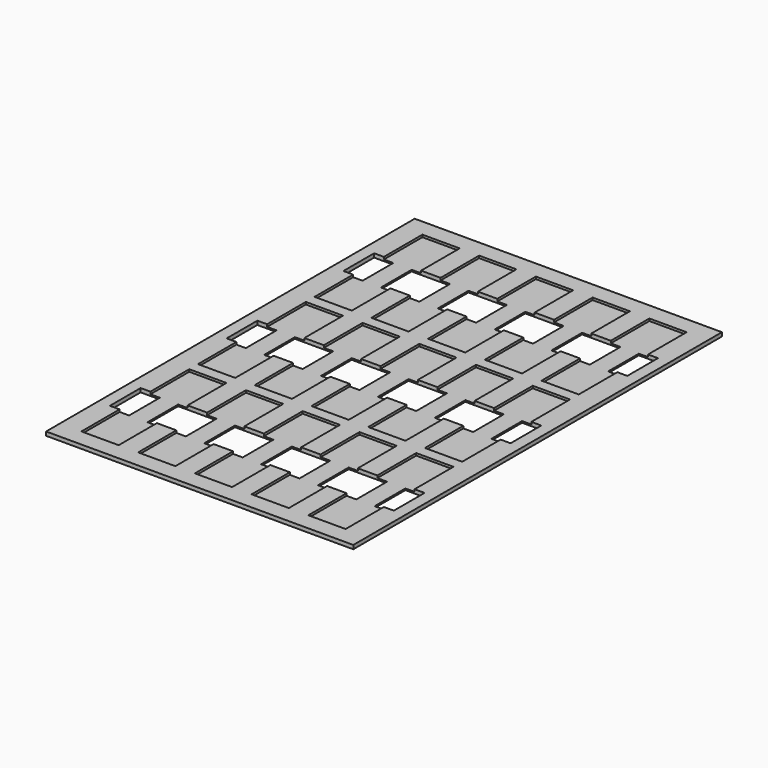
from build123d import *

# Parameters (mm, degrees)
F0_W         = 400
F0_H         = 600
F1_DEPTH     = 2
F2_W         = 400
F2_H         = 600
F2_W_2       = 48.5
F2_H_2       = 175.5
F3_DEPTH     = 3
F4_W         = 50
F4_H         = 50
F4_W_2       = 25
F5_DEPTH     = 25
F6_T         = 2
F6_T3_DEPTH  = 7
F6_T5_DEPTH  = 52.5
F6_T7_DEPTH  = 66.25
F6_T9_DEPTH  = 6
F6_T11_DEPTH = 52.5
F6_T13_DEPTH = 52.5
F6_T15_DEPTH = 52.5
F6_T17_DEPTH = 52.5
F6_T19_DEPTH = 9
F6_T21_DEPTH = 67.25
F6_T23_DEPTH = 66.5
F6_T25_DEPTH = 67
F6_T27_DEPTH = 66.75
F6_T29_DEPTH = 66.75


# Not quite as in the source:
# - a shell that OpenCascade refuses in one call is made with other operations: the cavity is built on its own and cut out


with BuildPart() as f1:
    # F0 (on Top) → F1 (new body)
    with BuildSketch(Plane.XY):
        Rectangle(F0_W, F0_H)
    extrude(amount=F1_DEPTH)

    # F2 (on face) → F3 (join)
    with BuildSketch(Plane.XY.offset(2)):
        Rectangle(F2_W, F2_H)
        with Locations((-147.75, -189.75)):
            Rectangle(F2_W_2, F2_H_2, mode=Mode.SUBTRACT)
        with Locations((-73.875, -189.75)):
            Rectangle(F2_W_2, F2_H_2, mode=Mode.SUBTRACT)
        with Locations((0, -189.75)):
            Rectangle(F2_W_2, F2_H_2, mode=Mode.SUBTRACT)
        with Locations((73.875, -189.75)):
            Rectangle(F2_W_2, F2_H_2, mode=Mode.SUBTRACT)
        with Locations((147.75, -189.75)):
            Rectangle(F2_W_2, F2_H_2, mode=Mode.SUBTRACT)
        with Locations((-147.75, 0)):
            Rectangle(F2_W_2, F2_H_2, mode=Mode.SUBTRACT)
        with Locations((-73.875, 0)):
            Rectangle(F2_W_2, F2_H_2, mode=Mode.SUBTRACT)
        with Locations((-147.75, 189.75)):
            Rectangle(F2_W_2, F2_H_2, mode=Mode.SUBTRACT)
        with Locations((-73.875, 189.75)):
            Rectangle(F2_W_2, F2_H_2, mode=Mode.SUBTRACT)
        Rectangle(F2_W_2, F2_H_2, mode=Mode.SUBTRACT)
        with Locations((73.875, 0)):
            Rectangle(F2_W_2, F2_H_2, mode=Mode.SUBTRACT)
        with Locations((147.75, 0)):
            Rectangle(F2_W_2, F2_H_2, mode=Mode.SUBTRACT)
        with Locations((0, 189.75)):
            Rectangle(F2_W_2, F2_H_2, mode=Mode.SUBTRACT)
        with Locations((73.875, 189.75)):
            Rectangle(F2_W_2, F2_H_2, mode=Mode.SUBTRACT)
        with Locations((147.75, 189.75)):
            Rectangle(F2_W_2, F2_H_2, mode=Mode.SUBTRACT)
    extrude(amount=F3_DEPTH)

    # F4 (on face) → F5 (cut)
    with BuildSketch(Plane.XY.offset(5)):
        with Locations((-110.8125, 189.75)):
            Rectangle(F4_W, F4_H)
        with Locations((-110.8125, -0.25)):
            Rectangle(F4_W, F4_H)
        with Locations((-110.8125, -190.25)):
            Rectangle(F4_W, F4_H)
        with Locations((-36.8125, 189.75)):
            Rectangle(F4_W, F4_H)
        with Locations((-36.8125, -0.25)):
            Rectangle(F4_W, F4_H)
        with Locations((-36.8125, -190.25)):
            Rectangle(F4_W, F4_H)
        with Locations((37.1875, 189.75)):
            Rectangle(F4_W, F4_H)
        with Locations((37.1875, -0.25)):
            Rectangle(F4_W, F4_H)
        with Locations((37.1875, -190.25)):
            Rectangle(F4_W, F4_H)
        with Locations((111.1875, 189.75)):
            Rectangle(F4_W, F4_H)
        with Locations((111.1875, -0.25)):
            Rectangle(F4_W, F4_H)
        with Locations((111.1875, -190.25)):
            Rectangle(F4_W, F4_H)
        with Locations((-172.1875, 189.75)):
            Rectangle(F4_W_2, F4_H)
        with Locations((-172.1875, -0.25)):
            Rectangle(F4_W_2, F4_H)
        with Locations((172.5, 189.75)):
            Rectangle(F4_W_2, F4_H)
        with Locations((172.5, -0.25)):
            Rectangle(F4_W_2, F4_H)
        with Locations((-172.1875, -190.25)):
            Rectangle(F4_W_2, F4_H)
        with Locations((172.5, -190.25)):
            Rectangle(F4_W_2, F4_H)
    extrude(amount=-F5_DEPTH, mode=Mode.SUBTRACT)

    # F6: shell of thickness 2, made by hand


with BuildPart() as f6_core1:
    # F6_t2: copy of F1
    add(f1.part)

    # the walls: a layer under each face that stays
    f6_faces = [f6_core1.faces().sort_by_distance(p)[0] for p in [
        (0, -300, 2.5),
        (-200, 0, 2.5),
        (-114.2857142857, -257.1428571429, 5),
        (200, 0, 2.5),
        (0, 300, 2.5),
        (-147.75, -277.5, 3.5),
        (-123.5, -246.375, 3.5),
        (-110.8125, -215.25, 2.5),
        (-98.125, -246.375, 3.5),
        (-73.875, -277.5, 3.5),
        (-49.625, -246.375, 3.5),
        (-36.8125, -215.25, 2.5),
        (-24.25, -246.375, 3.5),
        (0, -277.5, 3.5),
        (24.25, -246.375, 3.5),
        (37.1875, -215.25, 2.5),
        (49.625, -246.375, 3.5),
        (73.875, -277.5, 3.5),
        (98.125, -246.375, 3.5),
        (111.1875, -215.25, 2.5),
        (123.5, -246.375, 3.5),
        (147.75, -277.5, 3.5),
        (172, -246.375, 3.5),
        (172.5, -215.25, 2.5),
        (185, -190.25, 2.5),
        (172.5, -165.25, 2.5),
        (172, -133.625, 3.5),
        (147.75, -102, 3.5),
        (123.5, -133.625, 3.5),
        (111.1875, -165.25, 2.5),
        (98.125, -133.625, 3.5),
        (73.875, -102, 3.5),
        (49.625, -133.625, 3.5),
        (37.1875, -165.25, 2.5),
        (24.25, -133.625, 3.5),
        (0, -102, 3.5),
        (-24.25, -133.625, 3.5),
        (-36.8125, -165.25, 2.5),
        (-49.625, -133.625, 3.5),
        (-73.875, -102, 3.5),
        (-98.125, -133.625, 3.5),
        (-110.8125, -165.25, 2.5),
        (-123.5, -133.625, 3.5),
        (-147.75, -102, 3.5),
        (-172, -133.625, 3.5),
        (-172.1875, -165.25, 2.5),
        (-184.6875, -190.25, 2.5),
        (-172.1875, -215.25, 2.5),
        (-172, -246.375, 3.5),
        (-147.75, -87.75, 3.5),
        (-123.5, -56.5, 3.5),
        (-110.8125, -25.25, 2.5),
        (-98.125, -56.5, 3.5),
        (-73.875, -87.75, 3.5),
        (-49.625, -56.5, 3.5),
        (-36.8125, -25.25, 2.5),
        (-24.25, -56.5, 3.5),
        (0, -87.75, 3.5),
        (24.25, -56.5, 3.5),
        (37.1875, -25.25, 2.5),
        (49.625, -56.5, 3.5),
        (73.875, -87.75, 3.5),
        (98.125, -56.5, 3.5),
        (111.1875, -25.25, 2.5),
        (123.5, -56.5, 3.5),
        (147.75, -87.75, 3.5),
        (172, -56.5, 3.5),
        (172.5, -25.25, 2.5),
        (185, -0.25, 2.5),
        (172.5, 24.75, 2.5),
        (172, 56.25, 3.5),
        (147.75, 87.75, 3.5),
        (123.5, 56.25, 3.5),
        (111.1875, 24.75, 2.5),
        (98.125, 56.25, 3.5),
        (73.875, 87.75, 3.5),
        (49.625, 56.25, 3.5),
        (37.1875, 24.75, 2.5),
        (24.25, 56.25, 3.5),
        (0, 87.75, 3.5),
        (-24.25, 56.25, 3.5),
        (-36.8125, 24.75, 2.5),
        (-49.625, 56.25, 3.5),
        (-73.875, 87.75, 3.5),
        (-98.125, 56.25, 3.5),
        (-110.8125, 24.75, 2.5),
        (-123.5, 56.25, 3.5),
        (-147.75, 87.75, 3.5),
        (-172, 56.25, 3.5),
        (-172.1875, 24.75, 2.5),
        (-184.6875, -0.25, 2.5),
        (-172.1875, -25.25, 2.5),
        (-172, -56.5, 3.5),
        (-147.75, 102, 3.5),
        (-123.5, 133.375, 3.5),
        (-110.8125, 164.75, 2.5),
        (-98.125, 133.375, 3.5),
        (-73.875, 102, 3.5),
        (-49.625, 133.375, 3.5),
        (-36.8125, 164.75, 2.5),
        (-24.25, 133.375, 3.5),
        (0, 102, 3.5),
        (24.25, 133.375, 3.5),
        (37.1875, 164.75, 2.5),
        (49.625, 133.375, 3.5),
        (73.875, 102, 3.5),
        (98.125, 133.375, 3.5),
        (111.1875, 164.75, 2.5),
        (123.5, 133.375, 3.5),
        (147.75, 102, 3.5),
        (172, 133.375, 3.5),
        (172.5, 164.75, 2.5),
        (185, 189.75, 2.5),
        (172.5, 214.75, 2.5),
        (172, 246.125, 3.5),
        (147.75, 277.5, 3.5),
        (123.5, 246.125, 3.5),
        (111.1875, 214.75, 2.5),
        (98.125, 246.125, 3.5),
        (73.875, 277.5, 3.5),
        (49.625, 246.125, 3.5),
        (37.1875, 214.75, 2.5),
        (24.25, 246.125, 3.5),
        (0, 277.5, 3.5),
        (-24.25, 246.125, 3.5),
        (-36.8125, 214.75, 2.5),
        (-49.625, 246.125, 3.5),
        (-73.875, 277.5, 3.5),
        (-98.125, 246.125, 3.5),
        (-110.8125, 214.75, 2.5),
        (-123.5, 246.125, 3.5),
        (-147.75, 277.5, 3.5),
        (-172, 246.125, 3.5),
        (-172.1875, 214.75, 2.5),
        (-184.6875, 189.75, 2.5),
        (-172.1875, 164.75, 2.5),
        (-172, 133.375, 3.5),
        (-159.6875, -190.25, 1),
        (-85.8125, -190.25, 1),
        (-135.8125, -190.25, 1),
        (-11.8125, -190.25, 1),
        (-61.8125, -190.25, 1),
        (62.1875, -190.25, 1),
        (12.1875, -190.25, 1),
        (136.1875, -190.25, 1),
        (86.1875, -190.25, 1),
        (160, -190.25, 1),
        (-159.6875, -0.25, 1),
        (-85.8125, -0.25, 1),
        (-135.8125, -0.25, 1),
        (-11.8125, -0.25, 1),
        (-61.8125, -0.25, 1),
        (-159.6875, 189.75, 1),
        (-135.8125, 189.75, 1),
        (-85.8125, 189.75, 1),
        (-11.8125, 189.75, 1),
        (-61.8125, 189.75, 1),
        (62.1875, -0.25, 1),
        (12.1875, -0.25, 1),
        (136.1875, -0.25, 1),
        (86.1875, -0.25, 1),
        (160, -0.25, 1),
        (62.1875, 189.75, 1),
        (12.1875, 189.75, 1),
        (136.1875, 189.75, 1),
        (86.1875, 189.75, 1),
        (160, 189.75, 1),
        (-147.75, -189.75, 2),
        (-73.875, -189.75, 2),
        (0, -189.75, 2),
        (73.875, -189.75, 2),
        (147.75, -189.75, 2),
        (-147.75, 0, 2),
        (-73.875, 0, 2),
        (0, 0, 2),
        (73.875, 0, 2),
        (147.75, 0, 2),
        (-147.75, 189.75, 2),
        (-73.875, 189.75, 2),
        (0, 189.75, 2),
        (73.875, 189.75, 2),
        (147.75, 189.75, 2),
    ]]
    thicken(f6_faces, amount=-F6_T, mode=Mode.SUBTRACT)

    # F6_s4 → F6_t3 (cut)
    with BuildSketch(Plane.XY):
        Polygon((-123.52, -277.48), (-123.5, -279.5), (-121.5, -279.5), (-121.5, -277.5), align=None)
        Polygon((-171.98, -277.48), (-172, -279.5), (-174, -279.5), (-174, -277.5), align=None)
        Polygon((-98.105, -277.48), (-100.125, -277.5), (-100.125, -279.5), (-98.125, -279.5), align=None)
        Polygon((-49.645, -277.48), (-49.625, -279.5), (-47.625, -279.5), (-47.625, -277.5), align=None)
        Polygon((-24.23, -277.48), (-26.25, -277.5), (-26.25, -279.5), (-24.25, -279.5), align=None)
        Polygon((24.23, -277.48), (24.25, -279.5), (26.25, -279.5), (26.25, -277.5), align=None)
        Polygon((49.645, -277.48), (47.625, -277.5), (47.625, -279.5), (49.625, -279.5), align=None)
        Polygon((98.105, -277.48), (98.125, -279.5), (100.125, -279.5), (100.125, -277.5), align=None)
        Polygon((123.52, -277.48), (121.5, -277.5), (121.5, -279.5), (123.5, -279.5), align=None)
        Polygon((171.98, -277.48), (172, -279.5), (174, -279.5), (174, -277.5), align=None)
        Polygon((171.98, -102.02), (174, -102), (174, -100), (172, -100), align=None)
        Polygon((123.52, -102.02), (123.5, -100), (121.5, -100), (121.5, -102), align=None)
        Polygon((98.105, -102.02), (100.125, -102), (100.125, -100), (98.125, -100), align=None)
        Polygon((49.645, -102.02), (49.625, -100), (47.625, -100), (47.625, -102), align=None)
        Polygon((24.23, -102.02), (26.25, -102), (26.25, -100), (24.25, -100), align=None)
        Polygon((-24.23, -102.02), (-24.25, -100), (-26.25, -100), (-26.25, -102), align=None)
        Polygon((-49.645, -102.02), (-47.625, -102), (-47.625, -100), (-49.625, -100), align=None)
        Polygon((-98.105, -102.02), (-98.125, -100), (-100.125, -100), (-100.125, -102), align=None)
        Polygon((-123.52, -102.02), (-121.5, -102), (-121.5, -100), (-123.5, -100), align=None)
        Polygon((-171.98, -102.02), (-172, -100), (-174, -100), (-174, -102), align=None)
        Polygon((-123.52, -87.73), (-123.5, -89.75), (-121.5, -89.75), (-121.5, -87.75), align=None)
        Polygon((-171.98, -87.73), (-172, -89.75), (-174, -89.75), (-174, -87.75), align=None)
        Polygon((-98.105, -87.73), (-100.125, -87.75), (-100.125, -89.75), (-98.125, -89.75), align=None)
        Polygon((-49.645, -87.73), (-49.625, -89.75), (-47.625, -89.75), (-47.625, -87.75), align=None)
        Polygon((-24.23, -87.73), (-26.25, -87.75), (-26.25, -89.75), (-24.25, -89.75), align=None)
        Polygon((24.23, -87.73), (24.25, -89.75), (26.25, -89.75), (26.25, -87.75), align=None)
        Polygon((49.645, -87.73), (47.625, -87.75), (47.625, -89.75), (49.625, -89.75), align=None)
        Polygon((98.105, -87.73), (98.125, -89.75), (100.125, -89.75), (100.125, -87.75), align=None)
        Polygon((123.52, -87.73), (121.5, -87.75), (121.5, -89.75), (123.5, -89.75), align=None)
        Polygon((171.98, -87.73), (172, -89.75), (174, -89.75), (174, -87.75), align=None)
        Polygon((171.98, 87.73), (174, 87.75), (174, 89.75), (172, 89.75), align=None)
        Polygon((123.52, 87.73), (123.5, 89.75), (121.5, 89.75), (121.5, 87.75), align=None)
        Polygon((98.105, 87.73), (100.125, 87.75), (100.125, 89.75), (98.125, 89.75), align=None)
        Polygon((49.645, 87.73), (49.625, 89.75), (47.625, 89.75), (47.625, 87.75), align=None)
        Polygon((24.23, 87.73), (26.25, 87.75), (26.25, 89.75), (24.25, 89.75), align=None)
        Polygon((-24.23, 87.73), (-24.25, 89.75), (-26.25, 89.75), (-26.25, 87.75), align=None)
        Polygon((-49.645, 87.73), (-47.625, 87.75), (-47.625, 89.75), (-49.625, 89.75), align=None)
        Polygon((-98.105, 87.73), (-98.125, 89.75), (-100.125, 89.75), (-100.125, 87.75), align=None)
        Polygon((-123.52, 87.73), (-121.5, 87.75), (-121.5, 89.75), (-123.5, 89.75), align=None)
        Polygon((-171.98, 87.73), (-172, 89.75), (-174, 89.75), (-174, 87.75), align=None)
        Polygon((-123.52, 102.02), (-123.5, 100), (-121.5, 100), (-121.5, 102), align=None)
        Polygon((-171.98, 102.02), (-172, 100), (-174, 100), (-174, 102), align=None)
        Polygon((-98.105, 102.02), (-100.125, 102), (-100.125, 100), (-98.125, 100), align=None)
        Polygon((-49.645, 102.02), (-49.625, 100), (-47.625, 100), (-47.625, 102), align=None)
        Polygon((-24.23, 102.02), (-26.25, 102), (-26.25, 100), (-24.25, 100), align=None)
        Polygon((24.23, 102.02), (24.25, 100), (26.25, 100), (26.25, 102), align=None)
        Polygon((49.645, 102.02), (47.625, 102), (47.625, 100), (49.625, 100), align=None)
        Polygon((98.105, 102.02), (98.125, 100), (100.125, 100), (100.125, 102), align=None)
        Polygon((123.52, 102.02), (121.5, 102), (121.5, 100), (123.5, 100), align=None)
        Polygon((171.98, 102.02), (172, 100), (174, 100), (174, 102), align=None)
        Polygon((171.98, 277.48), (174, 277.5), (174, 279.5), (172, 279.5), align=None)
        Polygon((123.52, 277.48), (123.5, 279.5), (121.5, 279.5), (121.5, 277.5), align=None)
        Polygon((98.105, 277.48), (100.125, 277.5), (100.125, 279.5), (98.125, 279.5), align=None)
        Polygon((49.645, 277.48), (49.625, 279.5), (47.625, 279.5), (47.625, 277.5), align=None)
        Polygon((24.23, 277.48), (26.25, 277.5), (26.25, 279.5), (24.25, 279.5), align=None)
        Polygon((-24.23, 277.48), (-24.25, 279.5), (-26.25, 279.5), (-26.25, 277.5), align=None)
        Polygon((-49.645, 277.48), (-47.625, 277.5), (-47.625, 279.5), (-49.625, 279.5), align=None)
        Polygon((-98.105, 277.48), (-98.125, 279.5), (-100.125, 279.5), (-100.125, 277.5), align=None)
        Polygon((-123.52, 277.48), (-121.5, 277.5), (-121.5, 279.5), (-123.5, 279.5), align=None)
        Polygon((-171.98, 277.48), (-172, 279.5), (-174, 279.5), (-174, 277.5), align=None)
    extrude(amount=F6_T3_DEPTH, mode=Mode.SUBTRACT)

    # F6_s6 → F6_t5 (cut)
    with BuildSketch(Plane.YZ.offset(-174)):
        Polygon((-277.48, 2.02), (-279.5, 2), (-279.5, 0), (-277.5, 0), align=None)
        Polygon((-102.02, 2.02), (-100, 2), (-100, 0), (-102, 0), align=None)
        Polygon((-87.73, 2.02), (-89.75, 2), (-89.75, 0), (-87.75, 0), align=None)
        Polygon((87.73, 2.02), (89.75, 2), (89.75, 0), (87.75, 0), align=None)
        Polygon((102.02, 2.02), (100, 2), (100, 0), (102, 0), align=None)
        Polygon((277.48, 2.02), (279.5, 2), (279.5, 0), (277.5, 0), align=None)
    extrude(amount=F6_T5_DEPTH, mode=Mode.SUBTRACT)

    # F6_s8 → F6_t7 (cut)
    with BuildSketch(Plane.XZ.offset(213.25)):
        Polygon((-123.52, 2.02), (-121.5, 2), (-121.5, 0), (-123.5, 0), align=None)
        Polygon((-98.105, 2.02), (-100.125, 2), (-100.125, 0), (-98.125, 0), align=None)
        Polygon((-49.645, 2.02), (-47.625, 2), (-47.625, 0), (-49.625, 0), align=None)
        Polygon((-24.23, 2.02), (-26.25, 2), (-26.25, 0), (-24.25, 0), align=None)
        Polygon((24.23, 2.02), (26.25, 2), (26.25, 0), (24.25, 0), align=None)
        Polygon((49.645, 2.02), (47.625, 2), (47.625, 0), (49.625, 0), align=None)
        Polygon((98.105, 2.02), (100.125, 2), (100.125, 0), (98.125, 0), align=None)
        Polygon((123.52, 2.02), (121.5, 2), (121.5, 0), (123.5, 0), align=None)
        Polygon((171.98, 2.02), (174, 2), (174, 0), (172, 0), align=None)
        Polygon((-171.98, 2.02), (-174, 2), (-174, 0), (-172, 0), align=None)
    extrude(amount=F6_T7_DEPTH, mode=Mode.SUBTRACT)

    # F6_s10 → F6_t9 (cut)
    with BuildSketch(Plane.XY.offset(-2)):
        Polygon((-85.8325, -215.23), (-85.8125, -217.25), (-83.8125, -217.25), (-83.8125, -215.25), align=None)
        Polygon((-135.7925, -215.23), (-135.8125, -217.25), (-137.8125, -217.25), (-137.8125, -215.25), align=None)
        Polygon((-11.8325, -215.23), (-11.8125, -217.25), (-9.8125, -217.25), (-9.8125, -215.25), align=None)
        Polygon((-61.7925, -215.23), (-61.8125, -217.25), (-63.8125, -217.25), (-63.8125, -215.25), align=None)
        Polygon((62.1675, -215.23), (62.1875, -217.25), (64.1875, -217.25), (64.1875, -215.25), align=None)
        Polygon((12.2075, -215.23), (12.1875, -217.25), (10.1875, -217.25), (10.1875, -215.25), align=None)
        Polygon((136.1675, -215.23), (136.1875, -217.25), (138.1875, -217.25), (138.1875, -215.25), align=None)
        Polygon((86.2075, -215.23), (86.1875, -217.25), (84.1875, -217.25), (84.1875, -215.25), align=None)
        Polygon((160.02, -215.23), (160, -217.25), (158, -217.25), (158, -215.25), align=None)
        Polygon((160.02, -165.27), (160, -163.25), (158, -163.25), (158, -165.25), align=None)
        Polygon((86.2075, -165.27), (86.1875, -163.25), (84.1875, -163.25), (84.1875, -165.25), align=None)
        Polygon((136.1675, -165.27), (136.1875, -163.25), (138.1875, -163.25), (138.1875, -165.25), align=None)
        Polygon((12.2075, -165.27), (12.1875, -163.25), (10.1875, -163.25), (10.1875, -165.25), align=None)
        Polygon((62.1675, -165.27), (62.1875, -163.25), (64.1875, -163.25), (64.1875, -165.25), align=None)
        Polygon((-61.7925, -165.27), (-61.8125, -163.25), (-63.8125, -163.25), (-63.8125, -165.25), align=None)
        Polygon((-11.8325, -165.27), (-11.8125, -163.25), (-9.8125, -163.25), (-9.8125, -165.25), align=None)
        Polygon((-135.7925, -165.27), (-135.8125, -163.25), (-137.8125, -163.25), (-137.8125, -165.25), align=None)
        Polygon((-85.8325, -165.27), (-85.8125, -163.25), (-83.8125, -163.25), (-83.8125, -165.25), align=None)
        Polygon((-159.7075, -165.27), (-159.6875, -163.25), (-157.6875, -163.25), (-157.6875, -165.25), align=None)
        Polygon((-159.7075, -215.23), (-159.6875, -217.25), (-157.6875, -217.25), (-157.6875, -215.25), align=None)
        Polygon((-85.8325, -25.23), (-85.8125, -27.25), (-83.8125, -27.25), (-83.8125, -25.25), align=None)
        Polygon((-135.7925, -25.23), (-135.8125, -27.25), (-137.8125, -27.25), (-137.8125, -25.25), align=None)
        Polygon((-11.8325, -25.23), (-11.8125, -27.25), (-9.8125, -27.25), (-9.8125, -25.25), align=None)
        Polygon((-61.7925, -25.23), (-61.8125, -27.25), (-63.8125, -27.25), (-63.8125, -25.25), align=None)
        Polygon((62.1675, -25.23), (62.1875, -27.25), (64.1875, -27.25), (64.1875, -25.25), align=None)
        Polygon((12.2075, -25.23), (12.1875, -27.25), (10.1875, -27.25), (10.1875, -25.25), align=None)
        Polygon((136.1675, -25.23), (136.1875, -27.25), (138.1875, -27.25), (138.1875, -25.25), align=None)
        Polygon((86.2075, -25.23), (86.1875, -27.25), (84.1875, -27.25), (84.1875, -25.25), align=None)
        Polygon((160.02, -25.23), (160, -27.25), (158, -27.25), (158, -25.25), align=None)
        Polygon((160.02, 24.73), (160, 26.75), (158, 26.75), (158, 24.75), align=None)
        Polygon((86.2075, 24.73), (86.1875, 26.75), (84.1875, 26.75), (84.1875, 24.75), align=None)
        Polygon((136.1675, 24.73), (136.1875, 26.75), (138.1875, 26.75), (138.1875, 24.75), align=None)
        Polygon((12.2075, 24.73), (12.1875, 26.75), (10.1875, 26.75), (10.1875, 24.75), align=None)
        Polygon((62.1675, 24.73), (62.1875, 26.75), (64.1875, 26.75), (64.1875, 24.75), align=None)
        Polygon((-61.7925, 24.73), (-61.8125, 26.75), (-63.8125, 26.75), (-63.8125, 24.75), align=None)
        Polygon((-11.8325, 24.73), (-11.8125, 26.75), (-9.8125, 26.75), (-9.8125, 24.75), align=None)
        Polygon((-135.7925, 24.73), (-135.8125, 26.75), (-137.8125, 26.75), (-137.8125, 24.75), align=None)
        Polygon((-85.8325, 24.73), (-85.8125, 26.75), (-83.8125, 26.75), (-83.8125, 24.75), align=None)
        Polygon((-159.7075, 24.73), (-159.6875, 26.75), (-157.6875, 26.75), (-157.6875, 24.75), align=None)
        Polygon((-159.7075, -25.23), (-159.6875, -27.25), (-157.6875, -27.25), (-157.6875, -25.25), align=None)
        Polygon((-85.8325, 164.77), (-85.8125, 162.75), (-83.8125, 162.75), (-83.8125, 164.75), align=None)
        Polygon((-135.7925, 164.77), (-135.8125, 162.75), (-137.8125, 162.75), (-137.8125, 164.75), align=None)
        Polygon((-11.8325, 164.77), (-11.8125, 162.75), (-9.8125, 162.75), (-9.8125, 164.75), align=None)
        Polygon((-61.7925, 164.77), (-61.8125, 162.75), (-63.8125, 162.75), (-63.8125, 164.75), align=None)
        Polygon((62.1675, 164.77), (62.1875, 162.75), (64.1875, 162.75), (64.1875, 164.75), align=None)
        Polygon((12.2075, 164.77), (12.1875, 162.75), (10.1875, 162.75), (10.1875, 164.75), align=None)
        Polygon((136.1675, 164.77), (136.1875, 162.75), (138.1875, 162.75), (138.1875, 164.75), align=None)
        Polygon((86.2075, 164.77), (86.1875, 162.75), (84.1875, 162.75), (84.1875, 164.75), align=None)
        Polygon((160.02, 164.77), (160, 162.75), (158, 162.75), (158, 164.75), align=None)
        Polygon((160.02, 214.73), (160, 216.75), (158, 216.75), (158, 214.75), align=None)
        Polygon((86.2075, 214.73), (86.1875, 216.75), (84.1875, 216.75), (84.1875, 214.75), align=None)
        Polygon((136.1675, 214.73), (136.1875, 216.75), (138.1875, 216.75), (138.1875, 214.75), align=None)
        Polygon((12.2075, 214.73), (12.1875, 216.75), (10.1875, 216.75), (10.1875, 214.75), align=None)
        Polygon((62.1675, 214.73), (62.1875, 216.75), (64.1875, 216.75), (64.1875, 214.75), align=None)
        Polygon((-61.7925, 214.73), (-61.8125, 216.75), (-63.8125, 216.75), (-63.8125, 214.75), align=None)
        Polygon((-11.8325, 214.73), (-11.8125, 216.75), (-9.8125, 216.75), (-9.8125, 214.75), align=None)
        Polygon((-135.7925, 214.73), (-135.8125, 216.75), (-137.8125, 216.75), (-137.8125, 214.75), align=None)
        Polygon((-85.8325, 214.73), (-85.8125, 216.75), (-83.8125, 216.75), (-83.8125, 214.75), align=None)
        Polygon((-159.7075, 214.73), (-159.6875, 216.75), (-157.6875, 216.75), (-157.6875, 214.75), align=None)
        Polygon((-159.7075, 164.77), (-159.6875, 162.75), (-157.6875, 162.75), (-157.6875, 164.75), align=None)
    extrude(amount=F6_T9_DEPTH, mode=Mode.SUBTRACT)

    # F6_s12 → F6_t11 (cut)
    with BuildSketch(Plane.YZ.offset(-100.125)):
        Polygon((-277.48, 2.02), (-279.5, 2), (-279.5, 0), (-277.5, 0), align=None)
        Polygon((-102.02, 2.02), (-100, 2), (-100, 0), (-102, 0), align=None)
        Polygon((-87.73, 2.02), (-89.75, 2), (-89.75, 0), (-87.75, 0), align=None)
        Polygon((87.73, 2.02), (89.75, 2), (89.75, 0), (87.75, 0), align=None)
        Polygon((102.02, 2.02), (100, 2), (100, 0), (102, 0), align=None)
        Polygon((277.48, 2.02), (279.5, 2), (279.5, 0), (277.5, 0), align=None)
    extrude(amount=F6_T11_DEPTH, mode=Mode.SUBTRACT)

    # F6_s14 → F6_t13 (cut)
    with BuildSketch(Plane.YZ.offset(-26.25)):
        Polygon((-277.48, 2.02), (-279.5, 2), (-279.5, 0), (-277.5, 0), align=None)
        Polygon((-102.02, 2.02), (-100, 2), (-100, 0), (-102, 0), align=None)
        Polygon((-87.73, 2.02), (-89.75, 2), (-89.75, 0), (-87.75, 0), align=None)
        Polygon((87.73, 2.02), (89.75, 2), (89.75, 0), (87.75, 0), align=None)
        Polygon((102.02, 2.02), (100, 2), (100, 0), (102, 0), align=None)
        Polygon((277.48, 2.02), (279.5, 2), (279.5, 0), (277.5, 0), align=None)
    extrude(amount=F6_T13_DEPTH, mode=Mode.SUBTRACT)

    # F6_s16 → F6_t15 (cut)
    with BuildSketch(Plane.YZ.offset(47.625)):
        Polygon((-277.48, 2.02), (-279.5, 2), (-279.5, 0), (-277.5, 0), align=None)
        Polygon((-102.02, 2.02), (-100, 2), (-100, 0), (-102, 0), align=None)
        Polygon((-87.73, 2.02), (-89.75, 2), (-89.75, 0), (-87.75, 0), align=None)
        Polygon((87.73, 2.02), (89.75, 2), (89.75, 0), (87.75, 0), align=None)
        Polygon((102.02, 2.02), (100, 2), (100, 0), (102, 0), align=None)
        Polygon((277.48, 2.02), (279.5, 2), (279.5, 0), (277.5, 0), align=None)
    extrude(amount=F6_T15_DEPTH, mode=Mode.SUBTRACT)

    # F6_s18 → F6_t17 (cut)
    with BuildSketch(Plane.YZ.offset(121.5)):
        Polygon((-277.48, 2.02), (-279.5, 2), (-279.5, 0), (-277.5, 0), align=None)
        Polygon((-102.02, 2.02), (-100, 2), (-100, 0), (-102, 0), align=None)
        Polygon((-87.73, 2.02), (-89.75, 2), (-89.75, 0), (-87.75, 0), align=None)
        Polygon((87.73, 2.02), (89.75, 2), (89.75, 0), (87.75, 0), align=None)
        Polygon((102.02, 2.02), (100, 2), (100, 0), (102, 0), align=None)
        Polygon((277.48, 2.02), (279.5, 2), (279.5, 0), (277.5, 0), align=None)
    extrude(amount=F6_T17_DEPTH, mode=Mode.SUBTRACT)

    # F6_s20 → F6_t19 (cut)
    with BuildSketch(Plane.XY.offset(-2)):
        Polygon((184.98, -215.23), (185, -217.25), (187, -217.25), (187, -215.25), align=None)
        Polygon((184.98, -165.27), (187, -165.25), (187, -163.25), (185, -163.25), align=None)
        Polygon((-184.6675, -165.27), (-184.6875, -163.25), (-186.6875, -163.25), (-186.6875, -165.25), align=None)
        Polygon((-184.6675, -215.23), (-186.6875, -215.25), (-186.6875, -217.25), (-184.6875, -217.25), align=None)
        Polygon((184.98, -25.23), (185, -27.25), (187, -27.25), (187, -25.25), align=None)
        Polygon((184.98, 24.73), (187, 24.75), (187, 26.75), (185, 26.75), align=None)
        Polygon((-184.6675, 24.73), (-184.6875, 26.75), (-186.6875, 26.75), (-186.6875, 24.75), align=None)
        Polygon((-184.6675, -25.23), (-186.6875, -25.25), (-186.6875, -27.25), (-184.6875, -27.25), align=None)
        Polygon((184.98, 164.77), (185, 162.75), (187, 162.75), (187, 164.75), align=None)
        Polygon((184.98, 214.73), (187, 214.75), (187, 216.75), (185, 216.75), align=None)
        Polygon((-184.6675, 214.73), (-184.6875, 216.75), (-186.6875, 216.75), (-186.6875, 214.75), align=None)
        Polygon((-184.6675, 164.77), (-186.6875, 164.75), (-186.6875, 162.75), (-184.6875, 162.75), align=None)
    extrude(amount=F6_T19_DEPTH, mode=Mode.SUBTRACT)

    # F6_s22 → F6_t21 (cut)
    with BuildSketch(Plane.XZ.offset(100)):
        Polygon((171.98, 2.02), (174, 2), (174, 0), (172, 0), align=None)
        Polygon((123.52, 2.02), (121.5, 2), (121.5, 0), (123.5, 0), align=None)
        Polygon((98.105, 2.02), (100.125, 2), (100.125, 0), (98.125, 0), align=None)
        Polygon((49.645, 2.02), (47.625, 2), (47.625, 0), (49.625, 0), align=None)
        Polygon((24.23, 2.02), (26.25, 2), (26.25, 0), (24.25, 0), align=None)
        Polygon((-24.23, 2.02), (-26.25, 2), (-26.25, 0), (-24.25, 0), align=None)
        Polygon((-49.645, 2.02), (-47.625, 2), (-47.625, 0), (-49.625, 0), align=None)
        Polygon((-98.105, 2.02), (-100.125, 2), (-100.125, 0), (-98.125, 0), align=None)
        Polygon((-123.52, 2.02), (-121.5, 2), (-121.5, 0), (-123.5, 0), align=None)
        Polygon((-171.98, 2.02), (-174, 2), (-174, 0), (-172, 0), align=None)
    extrude(amount=F6_T21_DEPTH, mode=Mode.SUBTRACT)

    # F6_s24 → F6_t23 (cut)
    with BuildSketch(Plane.XZ.offset(23.25)):
        Polygon((-123.52, 2.02), (-121.5, 2), (-121.5, 0), (-123.5, 0), align=None)
        Polygon((-98.105, 2.02), (-100.125, 2), (-100.125, 0), (-98.125, 0), align=None)
        Polygon((-49.645, 2.02), (-47.625, 2), (-47.625, 0), (-49.625, 0), align=None)
        Polygon((-24.23, 2.02), (-26.25, 2), (-26.25, 0), (-24.25, 0), align=None)
        Polygon((24.23, 2.02), (26.25, 2), (26.25, 0), (24.25, 0), align=None)
        Polygon((49.645, 2.02), (47.625, 2), (47.625, 0), (49.625, 0), align=None)
        Polygon((98.105, 2.02), (100.125, 2), (100.125, 0), (98.125, 0), align=None)
        Polygon((123.52, 2.02), (121.5, 2), (121.5, 0), (123.5, 0), align=None)
        Polygon((171.98, 2.02), (174, 2), (174, 0), (172, 0), align=None)
        Polygon((-171.98, 2.02), (-174, 2), (-174, 0), (-172, 0), align=None)
    extrude(amount=F6_T23_DEPTH, mode=Mode.SUBTRACT)

    # F6_s26 → F6_t25 (cut)
    with BuildSketch(Plane.XZ.offset(-89.75)):
        Polygon((171.98, 2.02), (174, 2), (174, 0), (172, 0), align=None)
        Polygon((123.52, 2.02), (121.5, 2), (121.5, 0), (123.5, 0), align=None)
        Polygon((98.105, 2.02), (100.125, 2), (100.125, 0), (98.125, 0), align=None)
        Polygon((49.645, 2.02), (47.625, 2), (47.625, 0), (49.625, 0), align=None)
        Polygon((24.23, 2.02), (26.25, 2), (26.25, 0), (24.25, 0), align=None)
        Polygon((-24.23, 2.02), (-26.25, 2), (-26.25, 0), (-24.25, 0), align=None)
        Polygon((-49.645, 2.02), (-47.625, 2), (-47.625, 0), (-49.625, 0), align=None)
        Polygon((-98.105, 2.02), (-100.125, 2), (-100.125, 0), (-98.125, 0), align=None)
        Polygon((-123.52, 2.02), (-121.5, 2), (-121.5, 0), (-123.5, 0), align=None)
        Polygon((-171.98, 2.02), (-174, 2), (-174, 0), (-172, 0), align=None)
    extrude(amount=F6_T25_DEPTH, mode=Mode.SUBTRACT)

    # F6_s28 → F6_t27 (cut)
    with BuildSketch(Plane.XZ.offset(-166.75)):
        Polygon((-123.52, 2.02), (-121.5, 2), (-121.5, 0), (-123.5, 0), align=None)
        Polygon((-98.105, 2.02), (-100.125, 2), (-100.125, 0), (-98.125, 0), align=None)
        Polygon((-49.645, 2.02), (-47.625, 2), (-47.625, 0), (-49.625, 0), align=None)
        Polygon((-24.23, 2.02), (-26.25, 2), (-26.25, 0), (-24.25, 0), align=None)
        Polygon((24.23, 2.02), (26.25, 2), (26.25, 0), (24.25, 0), align=None)
        Polygon((49.645, 2.02), (47.625, 2), (47.625, 0), (49.625, 0), align=None)
        Polygon((98.105, 2.02), (100.125, 2), (100.125, 0), (98.125, 0), align=None)
        Polygon((123.52, 2.02), (121.5, 2), (121.5, 0), (123.5, 0), align=None)
        Polygon((171.98, 2.02), (174, 2), (174, 0), (172, 0), align=None)
        Polygon((-171.98, 2.02), (-174, 2), (-174, 0), (-172, 0), align=None)
    extrude(amount=F6_T27_DEPTH, mode=Mode.SUBTRACT)

    # F6_s30 → F6_t29 (cut)
    with BuildSketch(Plane.XZ.offset(-279.5)):
        Polygon((171.98, 2.02), (174, 2), (174, 0), (172, 0), align=None)
        Polygon((123.52, 2.02), (121.5, 2), (121.5, 0), (123.5, 0), align=None)
        Polygon((98.105, 2.02), (100.125, 2), (100.125, 0), (98.125, 0), align=None)
        Polygon((49.645, 2.02), (47.625, 2), (47.625, 0), (49.625, 0), align=None)
        Polygon((24.23, 2.02), (26.25, 2), (26.25, 0), (24.25, 0), align=None)
        Polygon((-24.23, 2.02), (-26.25, 2), (-26.25, 0), (-24.25, 0), align=None)
        Polygon((-49.645, 2.02), (-47.625, 2), (-47.625, 0), (-49.625, 0), align=None)
        Polygon((-98.105, 2.02), (-100.125, 2), (-100.125, 0), (-98.125, 0), align=None)
        Polygon((-123.52, 2.02), (-121.5, 2), (-121.5, 0), (-123.5, 0), align=None)
        Polygon((-171.98, 2.02), (-174, 2), (-174, 0), (-172, 0), align=None)
    extrude(amount=F6_T29_DEPTH, mode=Mode.SUBTRACT)


with BuildPart() as f1_1:
    add(f1.part)

    # what is left inside the walls is the cavity
    f6_cavity = [f6_core1.part.solids().sort_by_distance(p)[0] for p in [
        (0, -99.333333, 2.98),
    ]]
    add(f6_cavity, mode=Mode.SUBTRACT)


solid = f1_1.part
